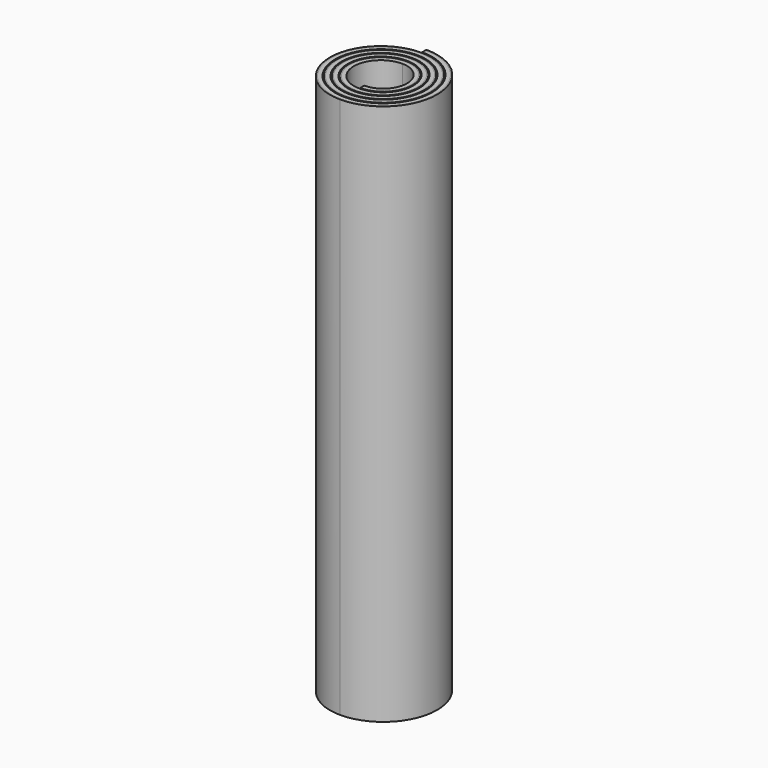
from build123d import *

# Parameters (mm, degrees)
F1_DEPTH = 610
F3_DEPTH = 610


# Not quite as in the source:
# - a feature of the source that left no trace in its solid (it failed there, or was rolled back) is left out


with BuildPart() as f1:
    # F0 (on Top) → F1 (new body)
    with BuildSketch(Plane.XY):
        with BuildLine():
            ThreePointArc((0, 28.5), (26.75, 1.75), (0, -25))
            Line((0, -25), (0, -29.399998486))
            ThreePointArc((0, -29.399998486), (31.149998486, 1.75), (0, 32.899998486))
            ThreePointArc((0, 32.899998486), (-34.649998486, -1.75), (0, -36.399998486))
            ThreePointArc((0, -36.399998486), (38.149998486, 1.75), (0, 39.899998486))
            ThreePointArc((0, 39.899998486), (-41.649998486, -1.75), (0, -43.399998486))
            ThreePointArc((0, -43.399998486), (45.149998486, 1.75), (0, 46.899998486))
            ThreePointArc((0, 46.899998486), (-48.649998486, -1.75), (0, -50.399998486))
            ThreePointArc((0, -50.399998486), (52.149998486, 1.75), (0, 53.899998486))
            ThreePointArc((0, 53.899998486), (-55.649998486, -1.75), (0, -57.399998486))
            ThreePointArc((0, -57.399998486), (59.149998486, 1.75), (0, 60.899998486))
            Line((0, 60.899998486), (0, 56.5))
            ThreePointArc((0, 56.5), (54.75, 1.75), (0, -53))
            ThreePointArc((0, -53), (-51.25, -1.75), (0, 49.5))
            ThreePointArc((0, 49.5), (47.75, 1.75), (0, -46))
            ThreePointArc((0, -46), (-44.25, -1.75), (0, 42.5))
            ThreePointArc((0, 42.5), (40.75, 1.75), (0, -39))
            ThreePointArc((0, -39), (-37.25, -1.75), (0, 35.5))
            ThreePointArc((0, 35.5), (33.75, 1.75), (0, -32))
            ThreePointArc((0, -32), (-30.25, -1.75), (0, 28.5))
        make_face()
    extrude(amount=F1_DEPTH)


with BuildPart() as f3:
    # F0 (on Top) → F3 (new body, through all)
    with BuildSketch(Plane.XY):
        with BuildLine():
            ThreePointArc((0, 32.899998486), (31.149998486, 1.75), (0, -29.399998486))
            Line((0, -29.399998486), (0, -30.899998486))
            ThreePointArc((0, -30.899998486), (32.649998486, 1.75), (0, 34.399998486))
            ThreePointArc((0, 34.399998486), (-36.149998486, -1.75), (0, -37.899998486))
            ThreePointArc((0, -37.899998486), (39.649998486, 1.75), (0, 41.399998486))
            ThreePointArc((0, 41.399998486), (-43.149998486, -1.75), (0, -44.899998486))
            ThreePointArc((0, -44.899998486), (46.649998486, 1.75), (0, 48.399998486))
            ThreePointArc((0, 48.399998486), (-50.149998486, -1.75), (0, -51.899998486))
            ThreePointArc((0, -51.899998486), (53.649998486, 1.75), (0, 55.399998486))
            ThreePointArc((0, 55.399998486), (-57.149998486, -1.75), (0, -58.899998486))
            ThreePointArc((0, -58.899998486), (60.649998486, 1.75), (0, 62.399998486))
            Line((0, 62.399998486), (0, 60.899998486))
            ThreePointArc((0, 60.899998486), (59.149998486, 1.75), (0, -57.399998486))
            ThreePointArc((0, -57.399998486), (-55.649998486, -1.75), (0, 53.899998486))
            ThreePointArc((0, 53.899998486), (52.149998486, 1.75), (0, -50.399998486))
            ThreePointArc((0, -50.399998486), (-48.649998486, -1.75), (0, 46.899998486))
            ThreePointArc((0, 46.899998486), (45.149998486, 1.75), (0, -43.399998486))
            ThreePointArc((0, -43.399998486), (-41.649998486, -1.75), (0, 39.899998486))
            ThreePointArc((0, 39.899998486), (38.149998486, 1.75), (0, -36.399998486))
            ThreePointArc((0, -36.399998486), (-34.649998486, -1.75), (0, 32.899998486))
        make_face()
    extrude(amount=F3_DEPTH)


solid = Compound([f1.part, f3.part])
